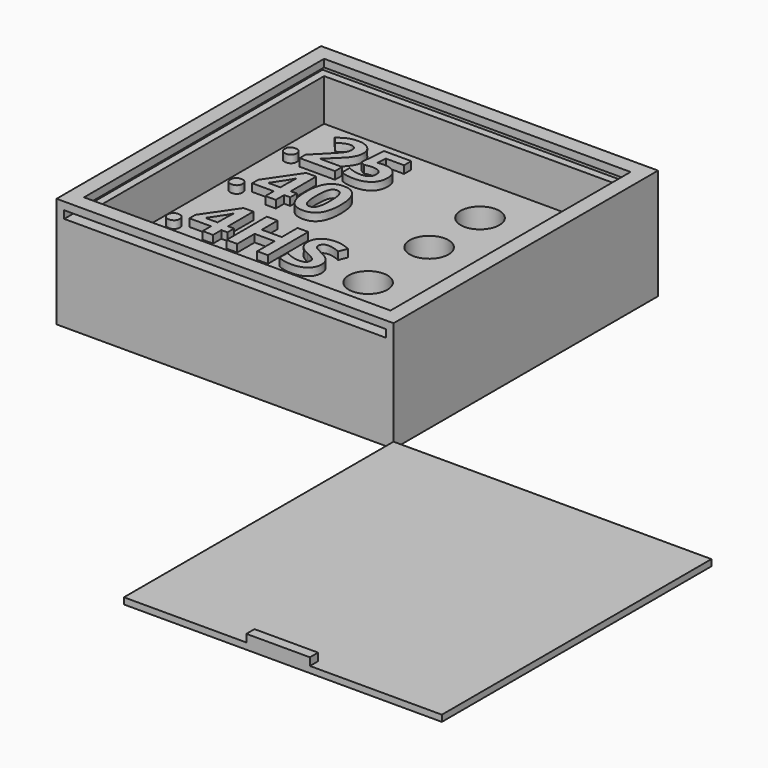
from build123d import *

# Parameters (mm, degrees)
F0_W         = 53
F0_H         = 52
F1_DEPTH     = 8.4
F2_R         = 3.05
F3_DEPTH     = 7
F2_TEXT_SIZE = 11.1111111111
F4_DEPTH     = 1.2
F5_W         = 53
F5_H         = 52
F5_W_2       = 48.2
F5_H_2       = 47.2
F6_DEPTH     = 9
F7_W         = 50.6
F7_H         = 1.2
F8_DEPTH     = 50.8
F9_W         = 50
F9_H         = 53
F10_DEPTH    = 1
F11_W        = 10
F11_H        = 1.6
F12_DEPTH    = 1.2


# Not quite as in the source:
# - Text() gives the source's letters only with a copy of the font that has no kerning and outlines rounded to 1/6400 em; it was checked with that copy


with BuildPart() as f1:
    # F0 (on Top) → F1 (new body)
    with BuildSketch(Plane.XY):
        with Locations((-26.5, 26)):
            Rectangle(F0_W, F0_H)
    extrude(amount=F1_DEPTH)

    # F2 (on face) → F3 (cut)
    with BuildSketch(Plane.XY.offset(8.4)):
        with Locations((-20, 42)):
            Circle(F2_R)
        with Locations((-10, 42)):
            Circle(F2_R)
        with Locations((-10, 32)):
            Circle(F2_R)
        with Locations((-20, 32)):
            Circle(F2_R)
        with Locations((-20, 20)):
            Circle(F2_R)
        with Locations((-10, 20)):
            Circle(F2_R)
        with Locations((-10, 10)):
            Circle(F2_R)
        with Locations((-20, 10)):
            Circle(F2_R)
    extrude(amount=-F3_DEPTH, mode=Mode.SUBTRACT)

    # F2 (on face) → F4 (join)
    with BuildSketch(Plane.XY.offset(8.4)):
        with Locations((-49.7261751376, 16.1900706589)):
            Text('.4HS', F2_TEXT_SIZE, font='Open Sans', font_style=FontStyle.BOLD, text_align=(TextAlign.LEFT, TextAlign.BOTTOM))
        with Locations((-49.5299212635, 28.287965253)):
            Text('.40', F2_TEXT_SIZE, font='Open Sans', font_style=FontStyle.BOLD, text_align=(TextAlign.LEFT, TextAlign.BOTTOM))
        with Locations((-49.4136113511, 38.8002060354)):
            Text('.25', F2_TEXT_SIZE, font='Open Sans', font_style=FontStyle.BOLD, text_align=(TextAlign.LEFT, TextAlign.BOTTOM))
    extrude(amount=F4_DEPTH)

    # F5 (on face) → F6 (join)
    with BuildSketch(Plane.XY.offset(8.4)):
        with Locations((-26.5, 26)):
            Rectangle(F5_W, F5_H)
        with Locations((-26.5, 26)):
            Rectangle(F5_W_2, F5_H_2, mode=Mode.SUBTRACT)
    extrude(amount=F6_DEPTH)

    # F7 (on face) → F8 (cut)
    with BuildSketch(Plane.XZ):
        with Locations((-26.5, 15.6)):
            Rectangle(F7_W, F7_H)
    extrude(amount=-F8_DEPTH, mode=Mode.SUBTRACT)


with BuildPart() as f10:
    # F9 (on Top) → F10 (new body)
    with BuildSketch(Plane.XY):
        with Locations((25, -26.5)):
            Rectangle(F9_W, F9_H)
    extrude(amount=F10_DEPTH)

    # F11 (on face) → F12 (join)
    with BuildSketch(Plane.XY.offset(1)):
        with Locations((24.2500501871, -52.2)):
            Rectangle(F11_W, F11_H)
    extrude(amount=F12_DEPTH)


solid = Compound([f1.part, f10.part])
